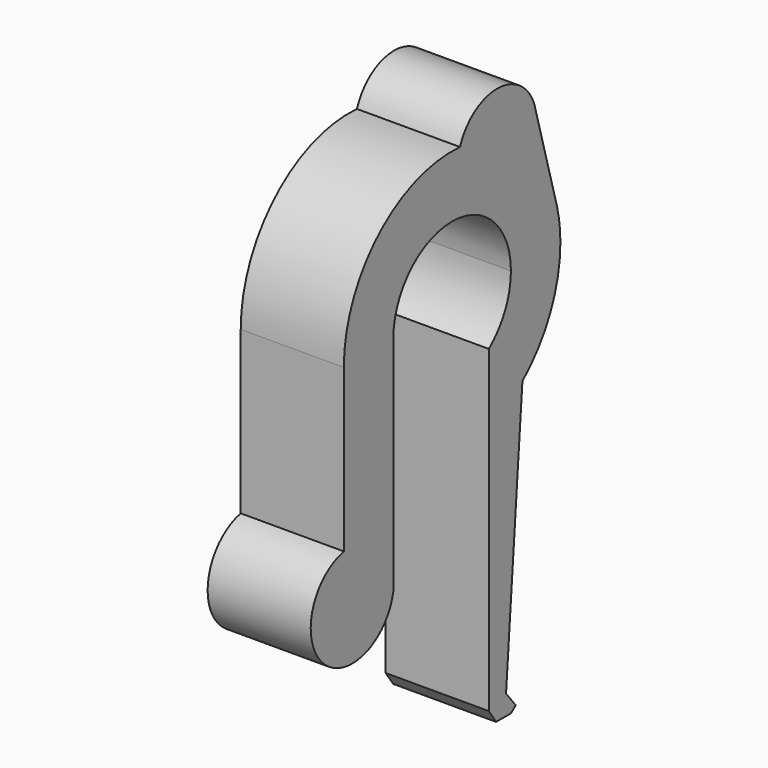
from build123d import *

# Parameters (mm, degrees)
F1_DEPTH = 25


# Not quite as in the source:
# - a feature names something its author has since deleted; it is built from what else it names


with BuildPart() as f1:
    # F0 (on Right) → F1 (new body)
    with BuildSketch(Plane.YZ):
        with BuildLine():
            Line((21.3200338185, 0), (17.8281293297, 0))
            ThreePointArc((17.8281293297, 0), (16.0680734174, -7.7239376), (11.135423556, -13.9228063846))
            Line((11.135423556, -13.9228063846), (11.135423556, -30.8818460833))
            ThreePointArc((11.135423556, -30.8818460833), (16.4953904054, -28.3828851715), (21.3200338185, -24.9628170138))
            Line((21.3200338185, -24.9628170138), (21.3200338185, 0))
        make_face()
        with BuildLine():
            ThreePointArc((-17.8281293297, 0), (0, 17.8281293297), (17.8281293297, 0))
            Line((17.8281293297, 0), (21.3200338185, 0))
            Line((21.3200338185, 0), (21.3200338185, -24.9628170138))
            ThreePointArc((21.3200338185, -24.9628170138), (29.8126055788, -13.7438940584), (32.8281293297, 0))
            ThreePointArc((32.8281293297, 0), (32.5773816899, 4.0497256101), (31.8289692891, 8.0375860357))
            Line((31.8289692891, 8.0375860357), (31.3856816717, 9.6241914615))
            ThreePointArc((31.3856816717, 9.6241914615), (28.3999929291, 16.4659186477), (23.9458348633, 22.4562478608))
            ThreePointArc((23.9458348633, 22.4562478608), (8.5005350475, 17.8111454186), (2.3973170077, 32.7404787144))
            ThreePointArc((2.3973170077, 32.7404787144), (-22.3493472221, 24.0456389815), (-32.8281293297, 0))
            Line((-32.8281293297, 0), (-17.8281293297, 0))
        make_face()
        with BuildLine():
            Line((-17.8281293297, -27.5652658229), (-17.8281293297, 0))
            Line((-17.8281293297, 0), (-32.8281293297, 0))
            ThreePointArc((-32.8281293297, 0), (-28.8353100436, -15.6911111771), (-17.8281293297, -27.5652658229))
        make_face()
        with BuildLine():
            Line((-17.8281293297, -49.2888468657), (-17.8281293297, -27.5652658229))
            ThreePointArc((-17.8281293297, -27.5652658229), (-28.8353100436, -15.6911111771), (-32.8281293297, 0))
            Line((-32.8281293297, 0), (-32.8281293297, -39.2883635356))
            ThreePointArc((-32.8281293297, -39.2883635356), (-23.2296585262, -41.1410511261), (-17.8281293297, -49.2888468657))
        make_face()
        with BuildLine():
            ThreePointArc((21.3200338185, -24.9628170138), (16.4953904054, -28.3828851715), (11.135423556, -30.8818460833))
            Line((11.135423556, -30.8818460833), (11.135423556, -91.2536308169))
            Line((11.135423556, -91.2536308169), (16.2277286872, -91.2536308169))
            Line((16.2277286872, -91.2536308169), (16.3531204545, -89.621300844))
            Line((16.3531204545, -89.621300844), (21.3200338185, -24.9628170138))
        make_face()
        with BuildLine():
            Line((-17.8281293297, -49.3592731655), (-17.8281293297, -49.2888468657))
            ThreePointArc((-17.8281293297, -49.2888468657), (-23.2296585262, -41.1410511261), (-32.8281293297, -39.2883635356))
            Line((-32.8281293297, -39.2883635356), (-32.8281293297, -49.3592731655))
            Line((-32.8281293297, -49.3592731655), (-17.8281293297, -49.3592731655))
        make_face()
        with BuildLine():
            ThreePointArc((24.9010812958, 32.8337324859), (13.6167044371, 40.6286479576), (2.3973170077, 32.7404787144))
            ThreePointArc((2.3973170077, 32.7404787144), (14.1397228999, 29.626918699), (23.9458348633, 22.4562478608))
            ThreePointArc((23.9458348633, 22.4562478608), (25.2235009878, 25.4290316666), (25.6599794461, 28.6351758987))
            ThreePointArc((25.6599794461, 28.6351758987), (25.6074521104, 29.7564349958), (25.4503302031, 30.867872709))
            Line((25.4503302031, 30.867872709), (24.9010812958, 32.8337324859))
        make_face()
        with BuildLine():
            ThreePointArc((23.9458348633, 22.4562478608), (14.1397228999, 29.626918699), (2.3973170077, 32.7404787144))
            ThreePointArc((2.3973170077, 32.7404787144), (8.5005350475, 17.8111454186), (23.9458348633, 22.4562478608))
        make_face()
        with BuildLine():
            Line((-32.8281293297, -49.3592731655), (-32.8281293297, -39.2883635356))
            ThreePointArc((-32.8281293297, -39.2883635356), (-39.0840214493, -60.6643501174), (-17.8281293297, -54.0118288841))
            Line((-17.8281293297, -54.0118288841), (-17.8281293297, -49.3592731655))
            Line((-17.8281293297, -49.3592731655), (-32.8281293297, -49.3592731655))
        make_face()
        Polygon((16.2277286872, -91.2536308169), (11.135423556, -91.2536308169), (13.3315734565, -94.4593122868), (17.8637079006, -94.4593122868), (19.3015802652, -93.3099836111), (17.6578841403, -91.2536308169), align=None)
        Polygon((17.6578841403, -91.2536308169), (16.3531204545, -89.621300844), (16.2277286872, -91.2536308169), align=None)
        with BuildLine():
            ThreePointArc((25.6599794461, 28.6351758987), (25.2235009878, 25.4290316666), (23.9458348633, 22.4562478608))
            ThreePointArc((23.9458348633, 22.4562478608), (28.3999929291, 16.4659186477), (31.3856816717, 9.6241914615))
            Line((31.3856816717, 9.6241914615), (25.4503302031, 30.867872709))
            ThreePointArc((25.4503302031, 30.867872709), (25.6074521104, 29.7564349958), (25.6599794461, 28.6351758987))
        make_face()
        with BuildLine():
            Line((31.3856816717, 9.6241914615), (31.8289692891, 8.0375860357))
            ThreePointArc((31.8289692891, 8.0375860357), (31.6172793456, 8.8336697962), (31.3856816717, 9.6241914615))
        make_face()
    extrude(amount=F1_DEPTH)


solid = f1.part
